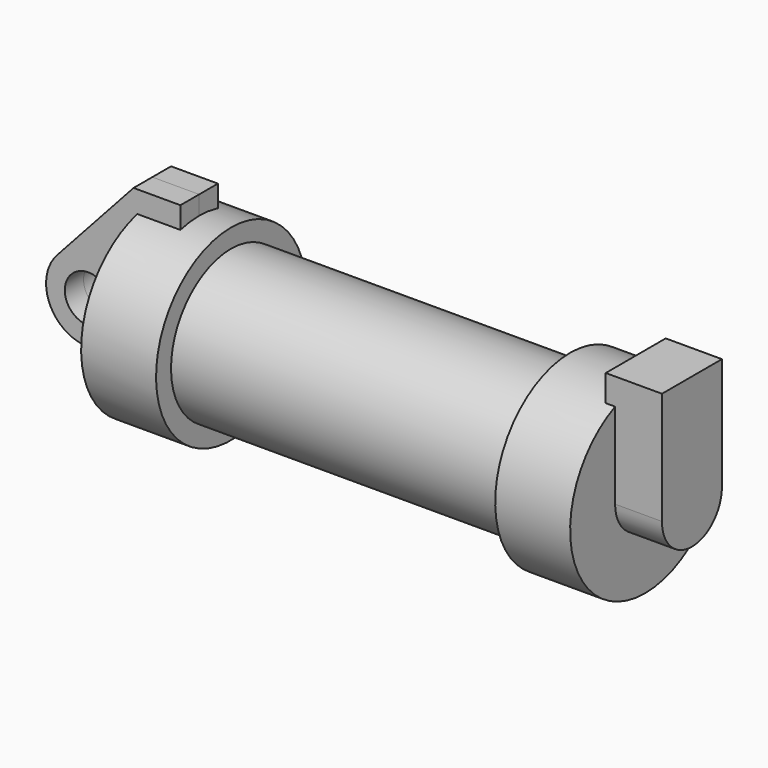
from build123d import *

# Parameters (mm, degrees)
F0_W          = 5.842
F0_H          = 12.7
F2_R          = 1.524
F3_DEPTH      = 6.35
F3_DEPTH_BACK = 1.27
F0_R          = 3.175
F5_DEPTH      = 3.175


# Not quite as in the source:
# - the program builds the solid bodies; features that only make, move or delete a surface that nothing else refers to are left out


with BuildPart() as f1:
    # F0 (on Front) → F1 (revolve)
    with BuildSketch(Plane.XZ):
        with Locations((2.921, 6.35)):
            Rectangle(F0_W, F0_H)
        Polygon((5.842, 12.7), (5.842, 0), (66.294, 0), (66.294, 12.7), (56.134, 12.7), (56.134, 10.16), (10.16, 10.16), (10.16, 12.7), align=None)
    revolve(axis=Axis((33.147, 0, 0), (-1, 0, 0)))

    # F2 (on face) → F3 (join, two sides)
    with BuildSketch(Plane.YZ.offset(66.294)) as f3_sk:
        with BuildLine():
            ThreePointArc((-5.08, 0), (0, 5.08), (5.08, 0))
            Line((5.08, 0), (5.08, 11.6397422652))
            ThreePointArc((5.08, 11.6397422652), (0, 12.7), (-5.08, 11.6397422652))
            Line((-5.08, 11.6397422652), (-5.08, 0))
        make_face()
        with BuildLine():
            ThreePointArc((-5.08, 11.6397422652), (0, 12.7), (5.08, 11.6397422652))
            Line((5.08, 11.6397422652), (5.08, 15.24))
            Line((5.08, 15.24), (-5.08, 15.24))
            Line((-5.08, 15.24), (-5.08, 11.6397422652))
        make_face()
        with BuildLine():
            ThreePointArc((-5.08, 0), (0, -5.08), (5.08, 0))
            ThreePointArc((5.08, 0), (0, 5.08), (-5.08, 0))
        make_face()
        Circle(F2_R, mode=Mode.SUBTRACT)
        Circle(F2_R)
    extrude(amount=F3_DEPTH)
    extrude(f3_sk.sketch, amount=-F3_DEPTH_BACK)


with BuildPart() as f5:
    # F0 (on Front) → F5 (new body, symmetric)
    with BuildSketch(Plane.XZ):
        with BuildLine():
            Line((-0.9398, 0), (0, 0))
            Line((0, 0), (0, 12.7))
            Line((0, 12.7), (5.842, 12.7))
            Line((5.842, 12.7), (5.842, 15.24))
            Line((5.842, 15.24), (-0.508, 15.24))
            Line((-0.508, 15.24), (-10.8806298187, 3.8475430269))
            ThreePointArc((-10.8806298187, 3.8475430269), (-4.5919612295, 5.3297205562), (-0.9398, 0))
        make_face()
        with BuildLine():
            ThreePointArc((-8.1826630726, -5.5069827884), (-3.1957909266, -4.5493385486), (-0.9398, 0))
            ThreePointArc((-0.9398, 0), (-4.5919612295, 5.3297205562), (-10.8806298187, 3.8475430269))
            ThreePointArc((-10.8806298187, 3.8475430269), (-12.1459778134, -1.5837270034), (-8.1826630726, -5.5069827884))
        make_face()
        with Locations((-6.6548, 0)):
            Circle(F0_R, mode=Mode.SUBTRACT)
        with Locations((2.921, 6.35)):
            Rectangle(F0_W, F0_H)
    extrude(amount=F5_DEPTH, both=True)


solid = Compound([f1.part, f5.part])
